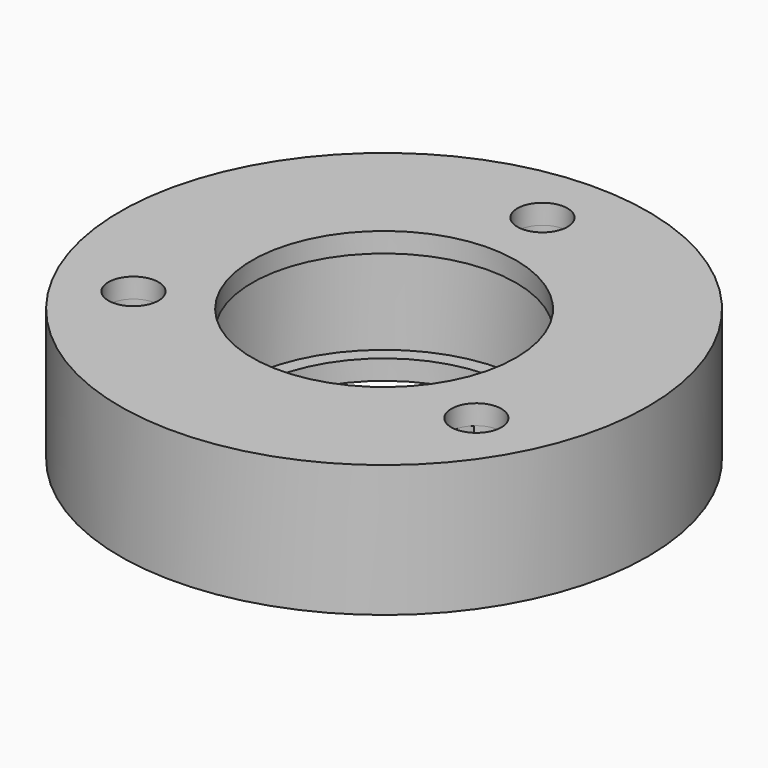
from build123d import *
from build123d import SkipClean  # not in build123d's __all__

# Parameters (mm, degrees)
F0_R     = 1.9
F0_R_2   = 10
F1_DEPTH = 1.5
F2_R     = 13.1
F2_R_2   = 11.1
F3_DEPTH = 7
F4_R     = 20
F5_DEPTH = 10
F6_R     = 19.4230477787
F6_R_2   = 1.9
F6_R_3   = 10
F7_DEPTH = 1.5
F9_DEPTH = 7


with BuildPart() as f1:
    # F0 (on Top) → F1 (new body)
    with BuildSketch(Plane.XY):
        with BuildLine():
            Line((-3.9, 15), (-3.9, 12.5059985607))
            ThreePointArc((-3.9, 12.5059985607), (-11.3449327896, 6.55), (-12.7805124532, -2.8755002056))
            Line((-12.7805124532, -2.8755002056), (-14.9403810568, -4.1225009252))
            ThreePointArc((-14.9403810568, -4.1225009252), (-16.3678801315, -9.45), (-11.0403810568, -10.8774990748))
            Line((-11.0403810568, -10.8774990748), (-8.8805124532, -9.6304983551))
            ThreePointArc((-8.8805124532, -9.6304983551), (0, -13.1), (8.8805124532, -9.6304983551))
            Line((8.8805124532, -9.6304983551), (11.0403810568, -10.8774990748))
            ThreePointArc((11.0403810568, -10.8774990748), (16.3678801315, -9.45), (14.9403810568, -4.1225009252))
            Line((14.9403810568, -4.1225009252), (12.7805124532, -2.8755002056))
            ThreePointArc((12.7805124532, -2.8755002056), (11.3449327896, 6.55), (3.9, 12.5059985607))
            Line((3.9, 12.5059985607), (3.9, 15))
            ThreePointArc((3.9, 15), (0, 18.9), (-3.9, 15))
        make_face()
        with Locations((-12.9903810568, -7.5)):
            Circle(F0_R, mode=Mode.SUBTRACT)
        with Locations((12.9903810568, -7.5)):
            Circle(F0_R, mode=Mode.SUBTRACT)
        Circle(F0_R_2, mode=Mode.SUBTRACT)
        with Locations((0, 15)):
            Circle(F0_R, mode=Mode.SUBTRACT)
    extrude(amount=-F1_DEPTH)

    # F2 (on face) → F3 (join)
    with BuildSketch(Plane.XY):
        Circle(F2_R)
        Circle(F2_R_2, mode=Mode.SUBTRACT)
    with SkipClean():  # cleaning this boolean's faces spoils the solid; the shape is the same uncleaned
        extrude(amount=F3_DEPTH)


with BuildPart() as f5:
    # F4 (on face) → F5 (new body)
    with BuildSketch(Plane(origin=(0, 0, -1.5), x_dir=(1, 0, 0), z_dir=(0, 0, -1))):
        Circle(F4_R)
        with BuildLine():
            ThreePointArc((12.8940350651, 2.8255724623), (13.1232858473, 1.4210448868), (13.2, 0))
            ThreePointArc((13.2, 0), (10.6545764815, -7.7923038955), (4, -12.5793481548))
            Line((4, -12.5793481548), (4, -15))
            ThreePointArc((4, -15), (0, -19), (-4, -15))
            Line((-4, -15), (-4, -12.5793481548))
            ThreePointArc((-4, -12.5793481548), (-11.43153533, -6.6), (-12.8940350651, 2.8255724623))
            Line((-12.8940350651, 2.8255724623), (-14.9903810568, 4.0358983849))
            ThreePointArc((-14.9903810568, 4.0358983849), (-16.4544826719, 9.5), (-10.9903810568, 10.9641016151))
            Line((-10.9903810568, 10.9641016151), (-8.8940350651, 9.7537756925))
            ThreePointArc((-8.8940350651, 9.7537756925), (0, 13.2), (8.8940350651, 9.7537756925))
            Line((8.8940350651, 9.7537756925), (10.9903810568, 10.9641016151))
            ThreePointArc((10.9903810568, 10.9641016151), (16.4544826719, 9.5), (14.9903810568, 4.0358983849))
            Line((14.9903810568, 4.0358983849), (12.8940350651, 2.8255724623))
        make_face(mode=Mode.SUBTRACT)
    extrude(amount=-F5_DEPTH)

    # F6 (on face) → F7 (join)
    with BuildSketch(Plane.XY.offset(8.5)):
        Circle(F6_R)
        with Locations((-12.9903810568, -7.5)):
            Circle(F6_R_2, mode=Mode.SUBTRACT)
        with Locations((12.9903810568, -7.5)):
            Circle(F6_R_2, mode=Mode.SUBTRACT)
        Circle(F6_R_3, mode=Mode.SUBTRACT)
        with Locations((0, 15)):
            Circle(F6_R_2, mode=Mode.SUBTRACT)
    extrude(amount=-F7_DEPTH)

    # F8 (on face) → F9 (join)
    with BuildSketch(Plane(origin=(0, 0, 7), x_dir=(1, 0, 0), z_dir=(0, 0, -1))):
        with BuildLine():
            Line((-14.9903810568, 4.0358983849), (-12.8940350651, 2.8255724623))
            ThreePointArc((-12.8940350651, 2.8255724623), (-12.4085336618, 4.5020320261), (-11.7060945509, 6.099782813))
            ThreePointArc((-11.7060945509, 6.099782813), (-14.635829324, 8.45), (-11.1356141491, 7.0878838537))
            ThreePointArc((-11.1356141491, 7.0878838537), (-10.1031409341, 8.4950893618), (-8.8940350651, 9.7537756925))
            Line((-8.8940350651, 9.7537756925), (-10.9903810568, 10.9641016151))
            ThreePointArc((-10.9903810568, 10.9641016151), (-16.4544826719, 9.5), (-14.9903810568, 4.0358983849))
        make_face()
        with BuildLine():
            ThreePointArc((-4, -15), (0, -19), (4, -15))
            Line((4, -15), (4, -12.5793481548))
            ThreePointArc((4, -12.5793481548), (2.3053927277, -12.9971213879), (0.5704804018, -13.1876666667))
            ThreePointArc((0.5704804018, -13.1876666667), (0, -16.9), (-0.5704804018, -13.1876666667))
            ThreePointArc((-0.5704804018, -13.1876666667), (-2.3053927277, -12.9971213879), (-4, -12.5793481548))
            Line((-4, -12.5793481548), (-4, -15))
        make_face()
        with BuildLine():
            ThreePointArc((14.9903810568, 4.0358983849), (16.4544826719, 9.5), (10.9903810568, 10.9641016151))
            Line((10.9903810568, 10.9641016151), (8.8940350651, 9.7537756925))
            ThreePointArc((8.8940350651, 9.7537756925), (10.1031409341, 8.4950893618), (11.1356141491, 7.0878838537))
            ThreePointArc((11.1356141491, 7.0878838537), (14.635829324, 8.45), (11.7060945509, 6.099782813))
            ThreePointArc((11.7060945509, 6.099782813), (12.4085336618, 4.5020320261), (12.8940350651, 2.8255724623))
            Line((12.8940350651, 2.8255724623), (14.9903810568, 4.0358983849))
        make_face()
    extrude(amount=F9_DEPTH)


solid = Compound([f1.part, f5.part])
